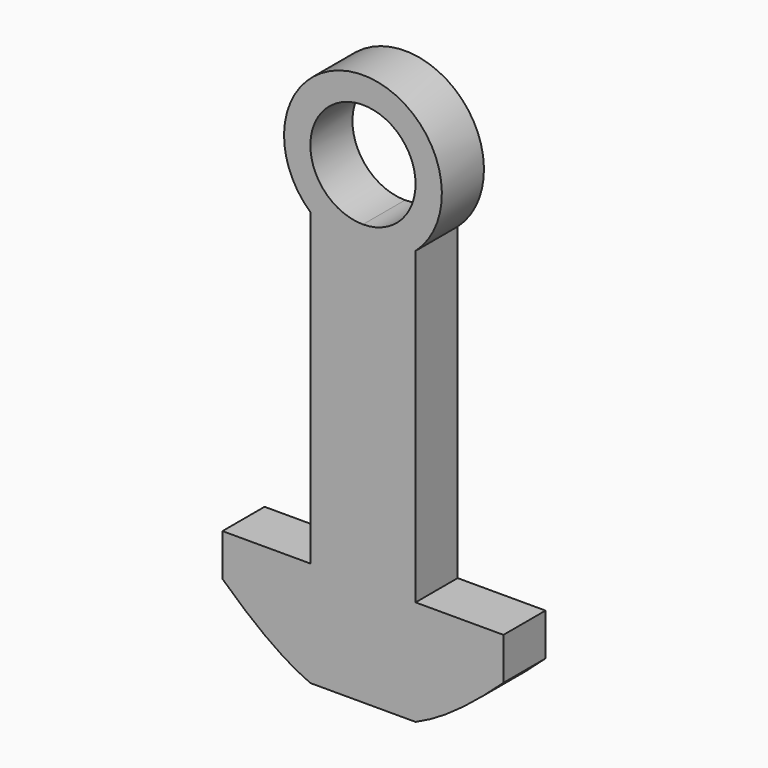
from build123d import *

# Parameters (mm, degrees)
F1_DEPTH      = 12.7
F3_DEPTH      = 19.05
F3_DEPTH_BACK = 19.05
F5_DEPTH      = 12.7


# Not quite as in the source:
# - a feature names something its author has since deleted; it is built from what else it names


with BuildPart() as f1:
    # F0 (on Front) → F1 (new body)
    with BuildSketch(Plane.XZ):
        with BuildLine():
            Line((-12.7, 0), (0, 0))
            Line((0, 0), (12.7, 0))
            Line((12.7, 0), (12.7, 49.3009683429))
            ThreePointArc((12.7, 49.3009683429), (0, 44.45), (-12.7, 49.3009683429))
            Line((-12.7, 49.3009683429), (-12.7, 0))
        make_face()
        Polygon((12.7, 0), (0, 0), (-12.7, 0), (-12.7, -25.4), (0, -25.4), (12.7, -25.4), align=None)
        with BuildLine():
            ThreePointArc((-12.7, 49.3009683429), (0, 44.45), (12.7, 49.3009683429))
            Line((12.7, 49.3009683429), (12.7, 50.8))
            Line((12.7, 50.8), (0, 50.8))
            Line((0, 50.8), (-12.7, 50.8))
            Line((-12.7, 50.8), (-12.7, 49.3009683429))
        make_face()
        with BuildLine():
            Line((12.7, 50.8), (12.7, 49.3009683429))
            ThreePointArc((12.7, 49.3009683429), (17.3901912008, 55.7228700667), (19.05, 63.5))
            ThreePointArc((19.05, 63.5), (13.4703841816, 76.9703841816), (0, 82.55))
            ThreePointArc((0, 82.55), (-17.7959834382, 70.2974608102), (-12.7, 49.3009683429))
            Line((-12.7, 49.3009683429), (-12.7, 50.8))
            Line((-12.7, 50.8), (0, 50.8))
            Line((0, 50.8), (12.7, 50.8))
        make_face()
        with BuildLine():
            ThreePointArc((12.7, 63.5), (8.9802561211, 54.5197438789), (0, 50.8))
            ThreePointArc((0, 50.8), (-8.9802561211, 72.4802561211), (12.7, 63.5))
        make_face(mode=Mode.SUBTRACT)
        with BuildLine():
            Line((33.9128470637, -25.4), (12.7, -25.4))
            Line((12.7, -25.4), (12.7, -50.8))
            add(Edge.make_bspline(
                [(12.7, -50.8), (19.8188597647, -47.7374133591), (26.8761157229, -42.0909685678), (33.9128470637, -35.5836565254)],
                knots=[0.6416254251, 0.6416254251, 0.6416254251, 0.6416254251, 0.8805998947, 0.8805998947, 0.8805998947, 0.8805998947], degree=3))
            Line((33.9128470637, -35.5836565254), (33.9128470637, -25.4))
        make_face()
        Polygon((12.7, -50.8), (12.7, -25.4), (0, -25.4), (-12.7, -25.4), (-12.7, -50.8), align=None)
        with BuildLine():
            Line((-12.7, -50.8), (-12.7, -25.4))
            Line((-12.7, -25.4), (-33.9128470637, -25.4))
            Line((-33.9128470637, -25.4), (-33.9128470637, -35.5836565254))
            add(Edge.make_bspline(
                [(-33.9128470637, -35.5836565254), (-26.8761157229, -42.0909685678), (-19.8188597647, -47.7374133591), (-12.7, -50.8)],
                knots=[0.1194001053, 0.1194001053, 0.1194001053, 0.1194001053, 0.3583745749, 0.3583745749, 0.3583745749, 0.3583745749], degree=3))
        make_face()
    extrude(amount=F1_DEPTH)

    # F2 (on Right) → F3 (cut, two sides)
    with BuildSketch(Plane.YZ) as f3_sk:
        Polygon((-7.62, -31.75), (-10.16, -31.75), (-10.16, -44.45), (-5.08, -44.45), (-2.54, -44.45), (-2.54, -31.75), (-5.08, -31.75), align=None)
    extrude(amount=-F3_DEPTH, mode=Mode.SUBTRACT)
    extrude(f3_sk.sketch, amount=F3_DEPTH_BACK, mode=Mode.SUBTRACT)

    # F4 (on face) → F5 (cut)
    with BuildSketch(Plane(origin=(0, 0, -50.8), x_dir=(1, 0, 0), z_dir=(0, 0, -1))):
        Polygon((-10.1655442268, 1.27), (0, 1.27), (10.16, 1.27), (10.16, 11.43), (0, 11.43), (-10.1655442268, 11.43), align=None)
    extrude(amount=-F5_DEPTH, mode=Mode.SUBTRACT)


solid = f1.part
